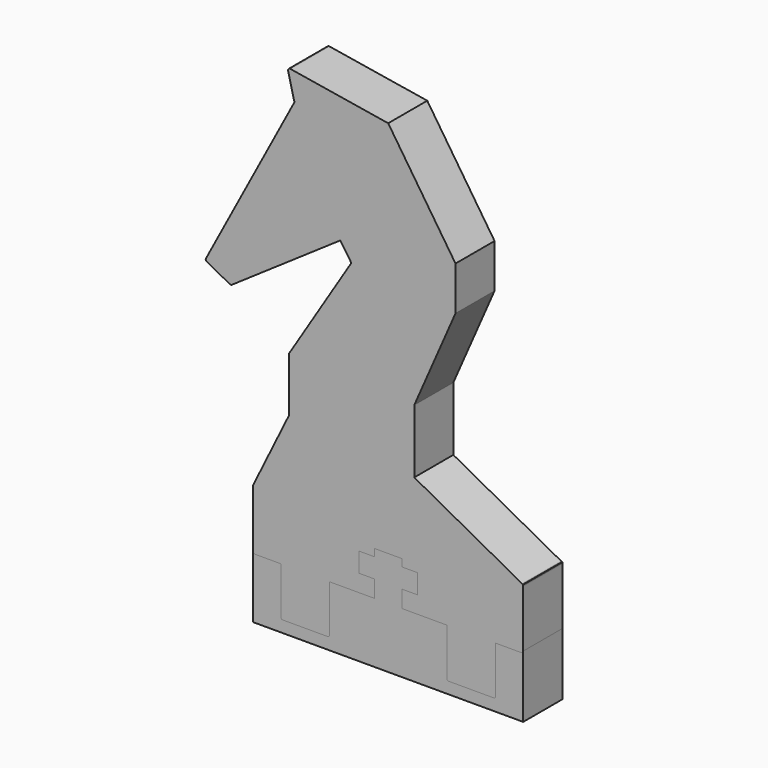
from build123d import *

# Parameters (mm, degrees)
F0_W     = 35.1139307306
F0_H     = 15.7079994678
F1_DEPTH = 6.35
F3_DEPTH = 6.35
F5_DEPTH = 25.4


with BuildPart() as f1:
    # F0 (on Front) → F1 (new body)
    with BuildSketch(Plane.XZ):
        Rectangle(F0_W, F0_H)
    extrude(amount=F1_DEPTH)


with BuildPart() as f3:
    # F2 (on face) → F3 (new body)
    with BuildSketch(Plane.XZ):
        with BuildLine():
            Line((-12.9048367962, 17.3293557018), (-17.5309673203, 7.9069519959))
            ThreePointArc((-17.5309673203, 7.9069519959), (-17.5419648563, 7.8810051625), (-17.5500203382, 7.8539997339))
            Line((-17.5500203382, 7.8539997339), (17.5070266734, 7.8539997339))
            ThreePointArc((17.5070266734, 7.8539997339), (17.4694564643, 7.8945796529), (17.4239940816, 7.9260665103))
            Line((17.4239940816, 7.9260665103), (3.3905450255, 15.5318096953))
            Line((3.3905450255, 15.5318096953), (3.3905450255, 23.8119002209))
            Line((3.3905450255, 23.8119002209), (8.7542133406, 36.0661039488))
            Line((8.7542133406, 36.0661039488), (8.7542133406, 41.7630597949))
            Line((8.7542133406, 41.7630597949), (0, 54.9788549542))
            Line((0, 54.9788549542), (-12.7324874569, 57.0608443233))
            ThreePointArc((-12.7324874569, 57.0608443233), (-12.9602708202, 56.9822894828), (-13.0199633728, 56.7488522906))
            Line((-13.0199633728, 56.7488522906), (-12.1920456474, 53.4209511994))
            Line((-12.1920456474, 53.4209511994), (-23.6994531811, 31.79702684))
            ThreePointArc((-23.6994531811, 31.79702684), (-23.7181539978, 31.6035252192), (-23.5945511638, 31.4534754366))
            Line((-23.5945511638, 31.4534754366), (-20.5967939678, 29.858186202))
            ThreePointArc((-20.5967939678, 29.858186202), (-20.4632994801, 29.8288084627), (-20.333908564, 29.8728745571))
            Line((-20.333908564, 29.8728745571), (-6.2368744391, 39.5311551932))
            Line((-6.2368744391, 39.5311551932), (-4.7932239249, 37.4240316451))
            Line((-4.7932239249, 37.4240316451), (-12.9048367962, 24.4077248131))
            Line((-12.9048367962, 24.4077248131), (-12.9048367962, 17.3293557018))
        make_face()
        with BuildLine():
            Line((17.5070266734, 7.8539997339), (-17.5500203382, 7.8539997339))
            ThreePointArc((-17.5500203382, 7.8539997339), (-17.5552231334, 7.8247083574), (-17.5569653653, 7.795009562))
            Line((-17.5569653653, 7.795009562), (-17.5569653653, 0.254))
            ThreePointArc((-17.5569653653, 0.254), (-17.4825704877, 0.0743948776), (-17.3029653653, 0))
            Line((-17.3029653653, 0), (-13.97, 0))
            Line((-13.97, 0), (-13.97, -6.096))
            ThreePointArc((-13.97, -6.096), (-13.8956051224, -6.2756051224), (-13.716, -6.35))
            Line((-13.716, -6.35), (-7.874, -6.35))
            ThreePointArc((-7.874, -6.35), (-7.6943948776, -6.2756051224), (-7.62, -6.096))
            Line((-7.62, -6.096), (-7.62, 0))
            Line((-7.62, 0), (7.62, 0))
            Line((7.62, 0), (7.62, -6.096))
            ThreePointArc((7.62, -6.096), (7.6943948776, -6.2756051224), (7.874, -6.35))
            Line((7.874, -6.35), (13.716, -6.35))
            ThreePointArc((13.716, -6.35), (13.8956051224, -6.2756051224), (13.97, -6.096))
            Line((13.97, -6.096), (13.97, 0))
            Line((13.97, 0), (17.3029653653, 0))
            ThreePointArc((17.3029653653, 0), (17.4825704877, 0.0743948776), (17.5569653653, 0.254))
            Line((17.5569653653, 0.254), (17.5569653653, 7.702754957))
            ThreePointArc((17.5569653653, 7.702754957), (17.5441577908, 7.7823929748), (17.5070266734, 7.8539997339))
        make_face()
    extrude(amount=F3_DEPTH)

    # F4 (on Front) → F5 (cut)
    with BuildSketch(Plane.XZ):
        Polygon((1.778, 5.715), (-1.778, 5.715), (-1.778, 4.7625), (-3.81, 4.7625), (-3.81, 2.2225), (-1.778, 2.2225), (-1.778, 0), (1.778, 0), (1.778, 2.2225), (3.81, 2.2225), (3.81, 4.7625), (1.778, 4.7625), align=None)
    extrude(amount=F5_DEPTH, mode=Mode.SUBTRACT)


solid = Compound([f1.part, f3.part])
